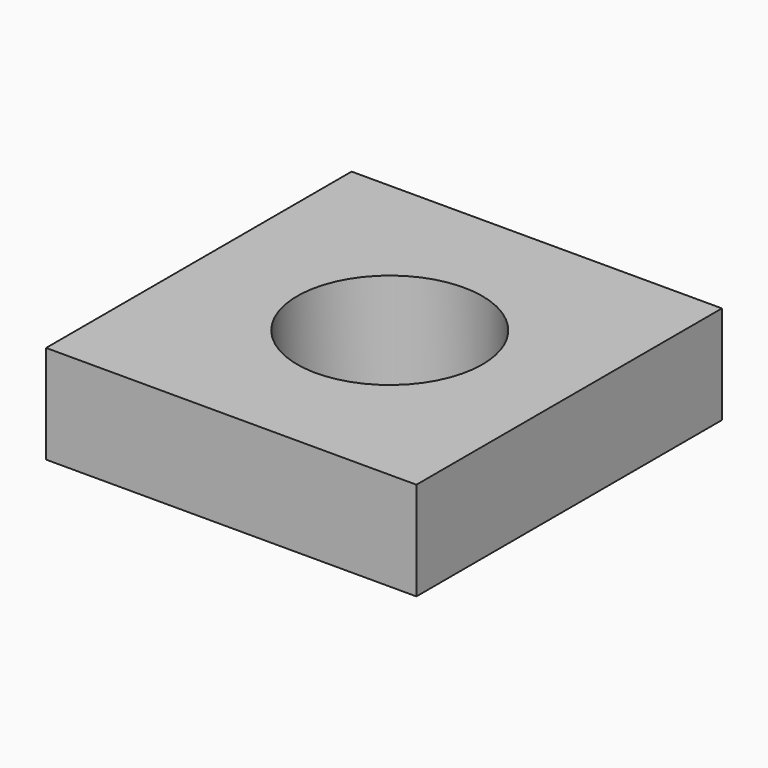
from build123d import *

# Parameters (mm, degrees)
F2_DEPTH = 50.8


# Not quite as in the source:
# - a variable given as a bare number and used for a length is read in inches; the dataset says mm whatever the document's units were


with BuildPart() as f2:
    # F1 (on Top) → F2 (new body)
    with BuildSketch(Plane.XY):
        Polygon((0, 98.61804), (-98.61804, 98.61804), (-98.61804, -98.61804), (92.65412, -98.61804), (92.65412, 98.61804), align=None)
        with BuildLine():
            ThreePointArc((47.81804, 0), (-46.2944321696, -11.9745772173), (41.82070094, 23.1860717313))
            ThreePointArc((41.82070094, 23.1860717313), (46.2944321696, 11.9745772173), (47.81804, 0))
        make_face(mode=Mode.SUBTRACT)
    extrude(amount=F2_DEPTH)


solid = f2.part
